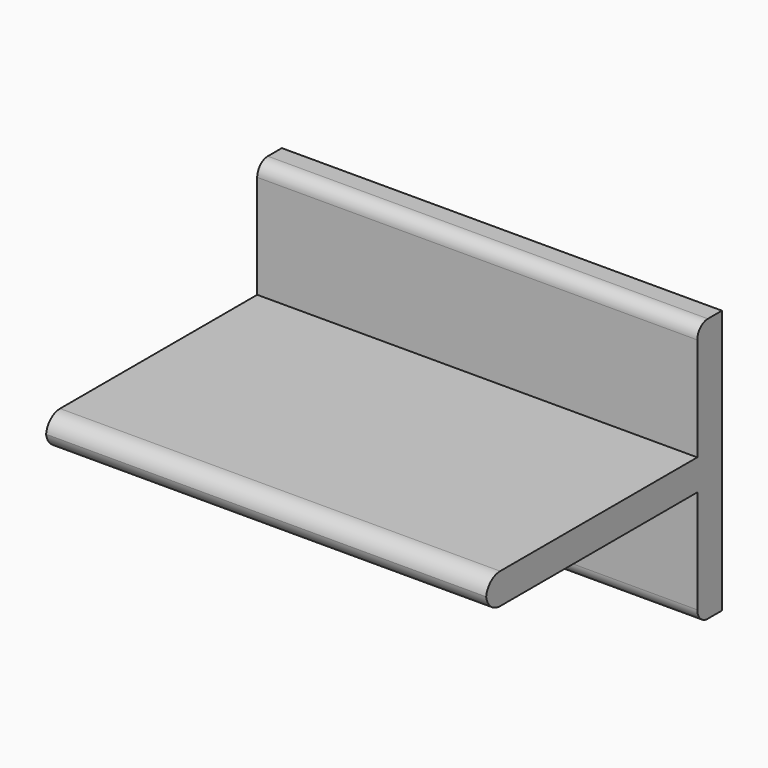
from build123d import *

# Parameters (mm, degrees)
F0_W        = 50
F0_H        = 30
F1_DEPTH    = 3.5
F2_R        = 1.5
F3_W        = 50
F3_H        = 3.5
F4_DEPTH    = 30
F5_T1_DEPTH = 60


# Not quite as in the source:
# - a fillet or chamfer that OpenCascade refuses, or shapes differently, is made with other operations: its cross-section is extruded or revolved along the edge and cut away or added


with BuildPart() as f1:
    # F0 (on Front) → F1 (new body)
    with BuildSketch(Plane.XZ):
        Rectangle(F0_W, F0_H)
    extrude(amount=F1_DEPTH)

    # F2
    f2_edges = [f1.edges().sort_by_distance(p)[0] for p in [
        (0, -3.5, 15),
        (0, -3.5, -15),
    ]]
    fillet(f2_edges, radius=F2_R)

    # F3 (on face) → F4 (join)
    with BuildSketch(Plane.XZ.offset(3.5)):
        Rectangle(F3_W, F3_H)
    extrude(amount=F4_DEPTH)

    # F5: fillet of radius 2 on 2 edges, made by hand

    # F5_s2 → F5_t1 (cut)
    with BuildSketch(Plane.YZ.offset(-30)):
        with BuildLine():
            ThreePointArc((-31.5, -1.75), (-32.9142135624, -1.1642135624), (-33.5, 0.25))
            Line((-33.5, 0.25), (-33.5, -1.75))
            Line((-33.5, -1.75), (-31.5, -1.75))
        make_face()
        with BuildLine():
            ThreePointArc((-31.5, 1.75), (-32.9142135624, 1.1642135624), (-33.5, -0.25))
            Line((-33.5, -0.25), (-33.5, 1.75))
            Line((-33.5, 1.75), (-31.5, 1.75))
        make_face()
    extrude(amount=F5_T1_DEPTH, mode=Mode.SUBTRACT)


solid = f1.part
